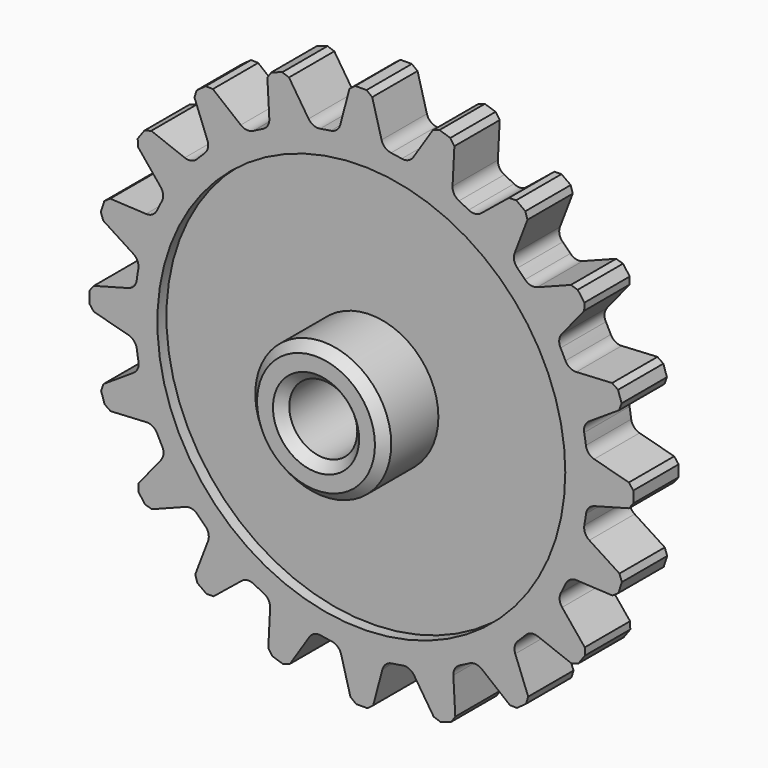
from build123d import *

# Parameters (mm, degrees)
F0_R            = 100
F2_DEPTH        = 25
F3_DEPTH        = 25
F3_COPIES_COUNT = 20
F4_R            = 5
F5_SIZE         = 2
F6_R            = 90
F7_DEPTH        = 5
F8_R            = 30
F9_DEPTH        = 30
F10_R           = 15
F11_DEPTH       = 50.001
F12_SIZE        = 4


# Not quite as in the source:
# - a pattern or mirror of a feature is missing from the dataset's text; its kind, count and spacing are read off the source's solid


with BuildPart() as f2:
    # F0 (on Front) → F2 (new body)
    with BuildSketch(Plane.XZ):
        Circle(F0_R)
    extrude(amount=F2_DEPTH)

    # F1 (on Front) → F3 (join, through all)
    with BuildSketch(Plane.XZ):
        Polygon((-10.1744222256, 99.4810591639), (9.8117977744, 99.5174789895), (4.281323162, 120.0080626686), (-4.7186618954, 119.9916624745), align=None)
    f3 = extrude(amount=F3_DEPTH)

    # F3_copies: F3 ×20 about axis
    f3_copies_axis = Axis((0, 0, 0), (0, 1, 0))
    for i in range(1, F3_COPIES_COUNT):
        add(f3.rotate(f3_copies_axis, i * 360 / F3_COPIES_COUNT))

    # F4
    f4_edges = [f2.edges().sort_by_distance(p)[0] for p in [
        (-10.174422, -12.5, 99.481059),
        (9.811798, -12.5, 99.517479),
        (-21.421018, -12.5, 97.678759),
        (97.678759, -12.5, 21.421018),
        (99.481059, -12.5, 10.174422),
        (99.517479, -12.5, -9.811798),
        (97.756179, -12.5, -21.064887),
        (91.614735, -12.5, -40.084166),
        (86.462243, -12.5, -50.242219),
        (74.744102, -12.5, -66.432818),
        (66.70478, -12.5, -74.501492),
        (50.556995, -12.5, -86.278562),
        (40.417788, -12.5, -91.46804),
        (21.421018, -12.5, -97.678759),
        (10.174422, -12.5, -99.481059),
        (-9.811798, -12.5, -99.517479),
        (-21.064887, -12.5, -97.756179),
        (-40.084166, -12.5, -91.614735),
        (-50.242219, -12.5, -86.462243),
        (-66.432818, -12.5, -74.744102),
        (-74.501492, -12.5, -66.70478),
        (-86.278562, -12.5, -50.556995),
        (-91.46804, -12.5, -40.417788),
        (-97.678759, -12.5, -21.421018),
        (-99.481059, -12.5, -10.174422),
        (-99.517479, -12.5, 9.811798),
        (-97.756179, -12.5, 21.064887),
        (-91.614735, -12.5, 40.084166),
        (-86.462243, -12.5, 50.242219),
        (-74.744102, -12.5, 66.432818),
        (-66.70478, -12.5, 74.501492),
        (-50.556995, -12.5, 86.278562),
        (-40.417788, -12.5, 91.46804),
        (21.064887, -12.5, 97.756179),
        (40.084166, -12.5, 91.614735),
        (50.242219, -12.5, 86.462243),
        (66.432818, -12.5, 74.744102),
        (74.501492, -12.5, 66.70478),
        (86.278562, -12.5, 50.556995),
        (91.46804, -12.5, 40.417788),
    ]]
    fillet(f4_edges, radius=F4_R)

    # F5
    f5_edges = [f2.edges().sort_by_distance(p)[0] for p in [
        (-4.718662, -12.5, 119.991662),
        (4.281323, -12.5, 120.008063),
        (115.457452, -12.5, 33.012751),
        (112.660706, -12.5, 41.567177),
        (119.991662, -12.5, 4.718662),
        (120.008063, -12.5, -4.281323),
        (99.605061, -12.5, 67.075306),
        (94.301734, -12.5, 74.346807),
        (115.576999, -12.5, -32.591749),
        (112.811448, -12.5, -41.156311),
        (74.002633, -12.5, 94.572064),
        (66.711852, -12.5, 99.848854),
        (99.848854, -12.5, -66.711852),
        (94.572064, -12.5, -74.002633),
        (41.156311, -12.5, 112.811448),
        (32.591749, -12.5, 115.576999),
        (74.346807, -12.5, -94.301734),
        (67.075306, -12.5, -99.605061),
        (41.567177, -12.5, -112.660706),
        (33.012751, -12.5, -115.457452),
        (-33.012751, -12.5, 115.457452),
        (-41.567177, -12.5, 112.660706),
        (4.718662, -12.5, -119.991662),
        (-4.281323, -12.5, -120.008063),
        (-67.075306, -12.5, 99.605061),
        (-74.346807, -12.5, 94.301734),
        (-32.591749, -12.5, -115.576999),
        (-41.156311, -12.5, -112.811448),
        (-94.572064, -12.5, 74.002633),
        (-99.848854, -12.5, 66.711852),
        (-66.711852, -12.5, -99.848854),
        (-74.002633, -12.5, -94.572064),
        (-112.811448, -12.5, 41.156311),
        (-115.576999, -12.5, 32.591749),
        (-94.301734, -12.5, -74.346807),
        (-99.605061, -12.5, -67.075306),
        (-120.008063, -12.5, 4.281323),
        (-119.991662, -12.5, -4.718662),
        (-112.660706, -12.5, -41.567177),
        (-115.457452, -12.5, -33.012751),
    ]]
    chamfer(f5_edges, length=F5_SIZE)

    # F6 (on face) → F7 (cut)
    with BuildSketch(Plane.XZ.offset(25)):
        Circle(F6_R)
    extrude(amount=-F7_DEPTH, mode=Mode.SUBTRACT)

    # F8 (on face) → F9 (join)
    with BuildSketch(Plane.XZ.offset(20)):
        Circle(F8_R)
    extrude(amount=F9_DEPTH)

    # F10 (on face) → F11 (cut, through all)
    with BuildSketch(Plane.XZ.offset(50)):
        Circle(F10_R)
    extrude(amount=-F11_DEPTH, mode=Mode.SUBTRACT)

    # F12
    f12_edges = [f2.edges().sort_by_distance(p)[0] for p in [
        (-30, -50, 0),
        (-15, -50, 0),
    ]]
    chamfer(f12_edges, length=F12_SIZE)


solid = f2.part
